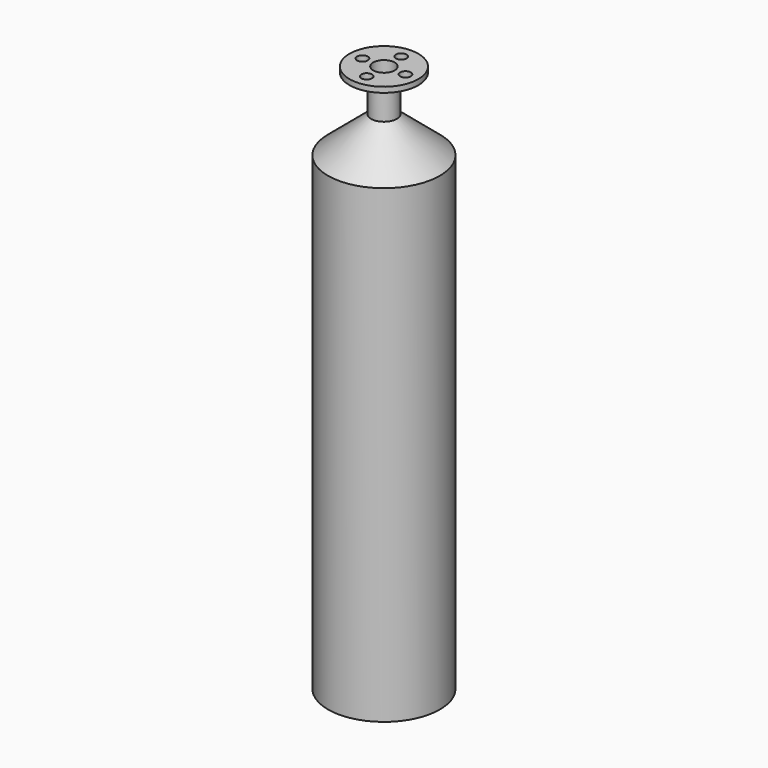
from build123d import *

# Parameters (mm, degrees)
F2_R     = 32
F2_R_2   = 12
F3_DEPTH = 5
F4_R     = 5
F5_DEPTH = 5


with BuildPart() as f1:
    # F0 (on Front) → F1 (revolve)
    with BuildSketch(Plane.XZ):
        Polygon((-50, 0), (-50, 434), (-10, 467.5639852471), (-10, 507.5639852471), (-12, 507.5639852471), (-12, 468.4966005634), (-52, 434.9326153163), (-52, -2), (0, -2), (0, 0), align=None)
    revolve(axis=Axis((0, 0, 216.0225092206), (0, 0, 1)))

    # F2 (on face) → F3 (join)
    with BuildSketch(Plane.XY.offset(507.5639852471)):
        Circle(F2_R)
        Circle(F2_R_2, mode=Mode.SUBTRACT)
    extrude(amount=-F3_DEPTH)

    # F4 (on face) → F5 (cut, through all)
    with BuildSketch(Plane.XY.offset(507.5639852471)):
        with Locations((0, 20)):
            Circle(F4_R)
        with Locations((-20, 0)):
            Circle(F4_R)
        with Locations((0, -20)):
            Circle(F4_R)
        with Locations((20, 0)):
            Circle(F4_R)
    extrude(amount=-F5_DEPTH, mode=Mode.SUBTRACT)


solid = f1.part
